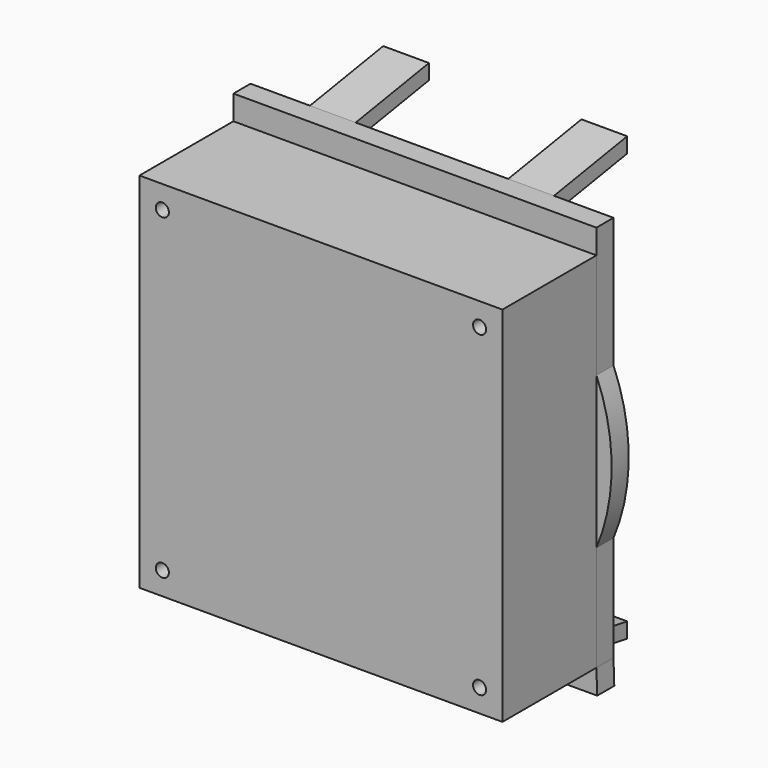
from build123d import *

# Parameters (mm, degrees)
F1_W     = 119
F1_H     = 119
F1_R     = 2.15
F2_DEPTH = 38.5
F3_R     = 2.15
F3_R_2   = 57.5
F4_DEPTH = 7
F6_START = 25
F6_DEPTH = 15


# Not quite as in the source:
# - a pattern or mirror of a feature is missing from the dataset's text; its kind, count and spacing are read off the source's solid


with BuildPart() as f2:
    # F1 (on Front) → F2 (new body)
    with BuildSketch(Plane.XZ):
        Rectangle(F1_W, F1_H)
        with Locations((-52, -52)):
            Circle(F1_R, mode=Mode.SUBTRACT)
        with Locations((52, -52)):
            Circle(F1_R, mode=Mode.SUBTRACT)
        with Locations((-52, 52)):
            Circle(F1_R, mode=Mode.SUBTRACT)
        with Locations((52, 52)):
            Circle(F1_R, mode=Mode.SUBTRACT)
    extrude(amount=F2_DEPTH)


with BuildPart() as f4:
    # F3 (on Front) → F4 (new body)
    with BuildSketch(Plane.XZ):
        with BuildLine():
            Line((59.7646775065, -67.5), (59.5, -59.5))
            Line((59.5, -59.5), (59.5, -24.899799196))
            ThreePointArc((59.5, -24.899799196), (64.5, 0), (59.5, 24.899799196))
            Line((59.5, 24.899799196), (59.5, 59.5))
            Line((59.5, 59.5), (59.5, 67.5))
            Line((59.5, 67.5), (-59.5, 67.5))
            Line((-59.5, 67.5), (-59.5, 59.5))
            Line((-59.5, 59.5), (-59.5, 24.899799196))
            ThreePointArc((-59.5, 24.899799196), (-64.5, 0), (-59.5, -24.899799196))
            Line((-59.5, -24.899799196), (-59.5, -59.5))
            Line((-59.5, -59.5), (-59.5, -67.5))
            Line((-59.5, -67.5), (59.7646775065, -67.5))
        make_face()
        with Locations((-52, -52)):
            Circle(F3_R, mode=Mode.SUBTRACT)
        with Locations((52, -52)):
            Circle(F3_R, mode=Mode.SUBTRACT)
        Circle(F3_R_2, mode=Mode.SUBTRACT)
        with Locations((-52, 52)):
            Circle(F3_R, mode=Mode.SUBTRACT)
        with Locations((52, 52)):
            Circle(F3_R, mode=Mode.SUBTRACT)
    extrude(amount=-F4_DEPTH)

    # F5 (on Right) → F6 (join)
    with BuildSketch(Plane.YZ.offset(F6_START)):
        Polygon((37, 72.5), (7, 67.5), (7, 62.5), (37, 67.5), align=None)
        Polygon((37, -67.5), (7, -62.5), (7, -67.5), (37, -72.5), align=None)
    f6 = extrude(amount=F6_DEPTH)

    # F6_copies: F6 across plane
    add(f6.mirror(Plane(origin=(0, 0, 0), x_dir=(0, 0, -1), z_dir=(-1, 0, 0))))


solid = Compound([f2.part, f4.part])
